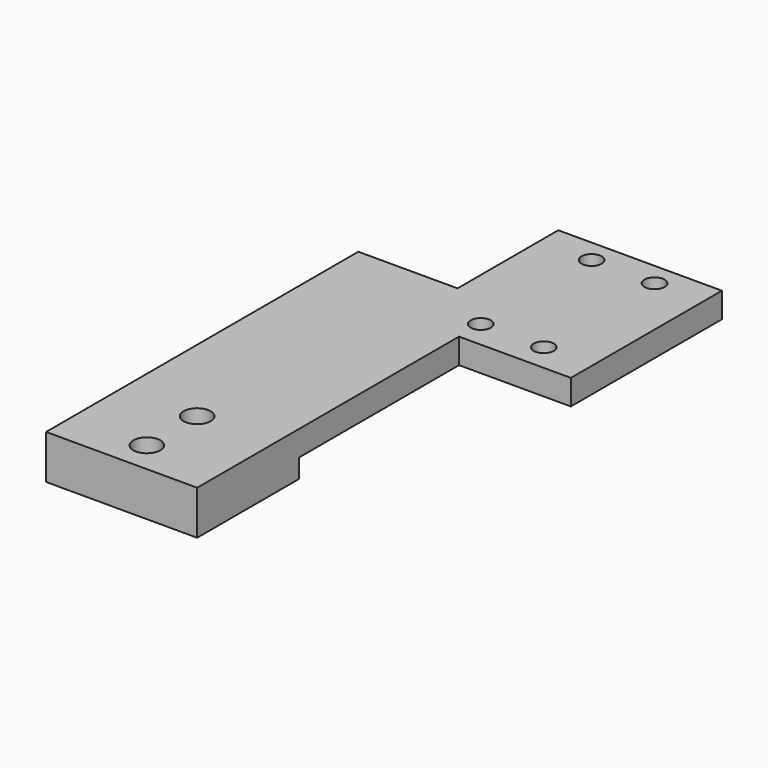
from build123d import *

# Parameters (mm, degrees)
F0_R     = 1.6
F0_W     = 24
F0_H     = 20.2417488769
F0_R_2   = 2.15
F1_DEPTH = 4
F2_DEPTH = 3


# Not quite as in the source:
# - a feature names something its author has since deleted; it is built from what else it names


with BuildPart() as f1:
    # F0 (on Top) → F1 (new body)
    with BuildSketch(Plane.XY):
        Polygon((-12, 47), (-12, 5.2417488769), (12, 5.2417488769), (12, 37), (29.7651190069, 37), (29.7651190069, 67), (3.7651190069, 67), (3.7651190069, 47), align=None)
        with Locations((12, 41.3295961916)):
            Circle(F0_R, mode=Mode.SUBTRACT)
        with Locations((22, 41.3295961916)):
            Circle(F0_R, mode=Mode.SUBTRACT)
        with Locations((12, 63.3295961916)):
            Circle(F0_R, mode=Mode.SUBTRACT)
        with Locations((22, 63.3295961916)):
            Circle(F0_R, mode=Mode.SUBTRACT)
        with Locations((0, -4.8791255616)):
            Rectangle(F0_W, F0_H)
        with Locations((0, -10)):
            Circle(F0_R_2, mode=Mode.SUBTRACT)
        Circle(F0_R_2, mode=Mode.SUBTRACT)
    extrude(amount=F1_DEPTH)

    # F0 (on Top) → F2 (join)
    with BuildSketch(Plane.XY):
        with Locations((0, -4.8791255616)):
            Rectangle(F0_W, F0_H)
        with Locations((0, -10)):
            Circle(F0_R_2, mode=Mode.SUBTRACT)
        Circle(F0_R_2, mode=Mode.SUBTRACT)
    extrude(amount=-F2_DEPTH)


solid = f1.part
